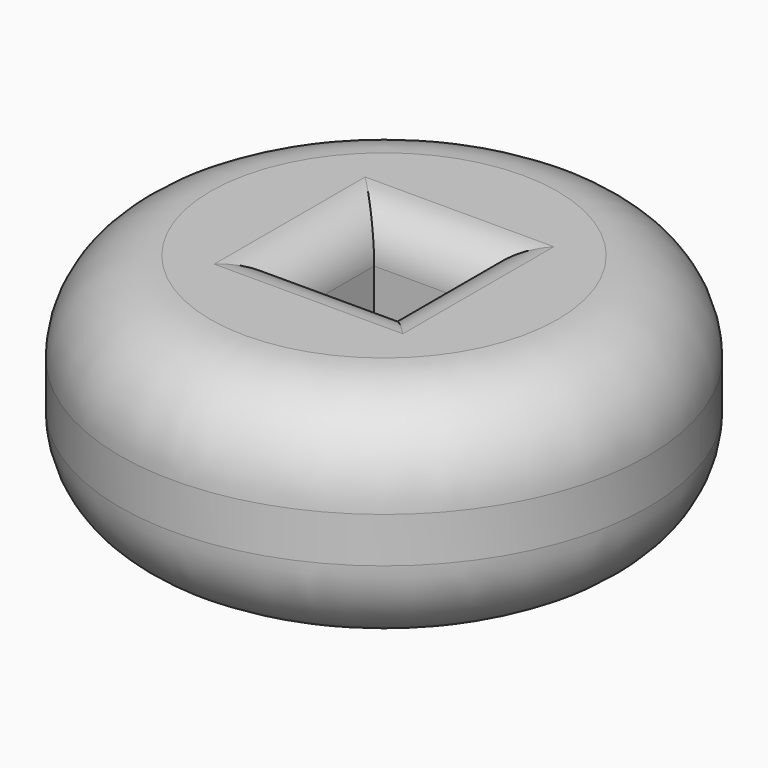
from build123d import *

# Parameters (mm, degrees)
F0_R     = 17.5
F0_W     = 6.5
F0_H     = 6.5
F1_DEPTH = 15
F2_R     = 6
F3_R     = 3


# Not quite as in the source:
# - a feature names something its author has since deleted; it is built from what else it names


with BuildPart() as f1:
    # F0 (on Top) → F1 (new body)
    with BuildSketch(Plane.XY):
        Circle(F0_R)
        Rectangle(F0_W, F0_H, mode=Mode.SUBTRACT)
    extrude(amount=F1_DEPTH)

    # F2
    f2_edges = [f1.edges().sort_by_distance(p)[0] for p in [
        (-17.5, 0, 15),
        (-17.5, 0, 0),
    ]]
    fillet(f2_edges, radius=F2_R)

    # F3
    f3_edges = [f1.edges().sort_by_distance(p)[0] for p in [
        (-3.25, 0, 15),
        (0, 3.25, 15),
        (3.25, 0, 15),
        (0, -3.25, 15),
        (0, 3.25, 0),
        (-3.25, 0, 0),
        (0, -3.25, 0),
        (3.25, 0, 0),
    ]]
    fillet(f3_edges, radius=F3_R)


solid = f1.part
